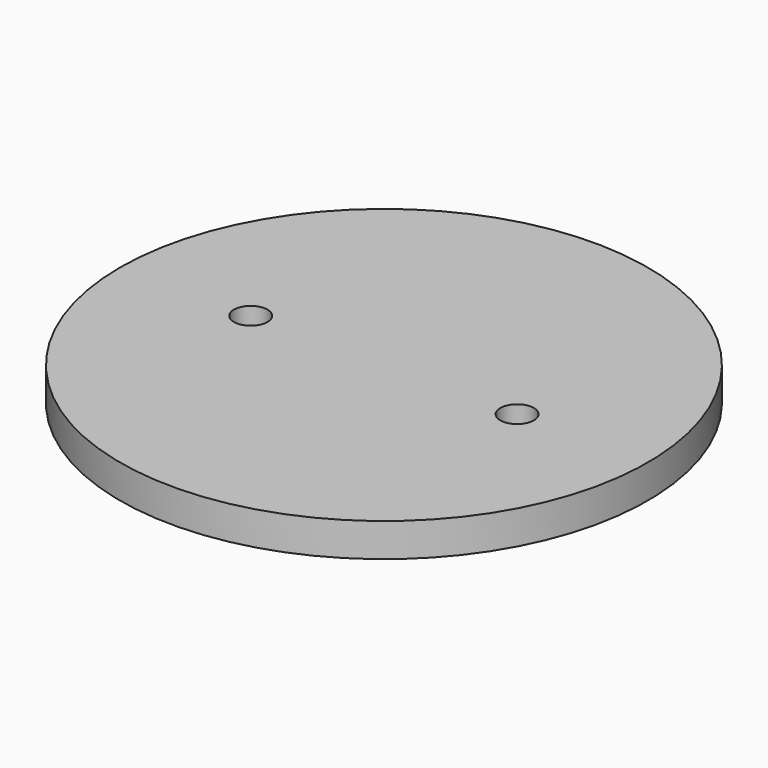
from build123d import *

# Parameters (mm, degrees)
F0_W = 49.55
F0_H = 6.3
F3_D = 6.3


# Not quite as in the source:
# - a feature names something its author has since deleted; it is built from what else it names


with BuildPart() as f1:
    # F0 (on Front) → F1 (revolve)
    with BuildSketch(Plane.XZ):
        with Locations((-24.775, 9.45)):
            Rectangle(F0_W, F0_H)
    revolve(axis=Axis((0, 0, -5.1516543608), (0, 0, -1)))

    # F3 (through all)
    with Locations(Plane(origin=(0, 0, 0), x_dir=(1, 0, 0), z_dir=(0, 0, -1))):
        with Locations((25, 0), (-25, 0)):
            Hole(F3_D / 2)


solid = f1.part
